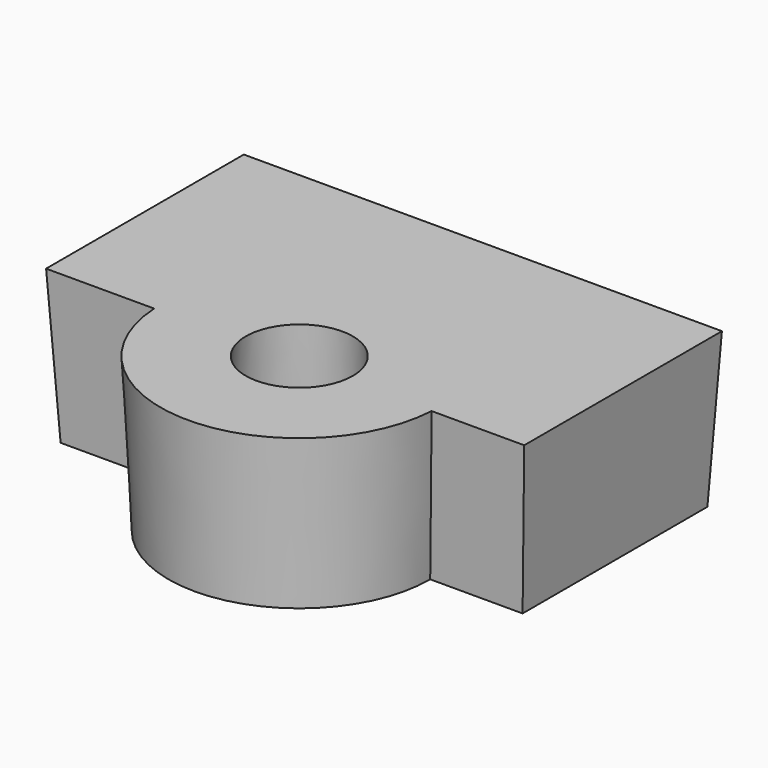
from build123d import *

# Parameters (mm, degrees)
F0_R                   = 10.16
F1_DEPTH               = 25.4
DRAFT_F1_DRAFTED_ANGLE = -3


# Not quite as in the source:
# - an extrude with a draft is written as a straight extrude whose walls are then drafted


with BuildPart() as f1:
    # F0 (on Top) → F1 (new body)
    with BuildSketch(Plane.XY):
        with BuildLine():
            Line((40.546802333, 18.3483660635), (-35.653197667, 18.3483660635))
            Line((-35.653197667, 18.3483660635), (-35.653197667, -19.7516339365))
            Line((-35.653197667, -19.7516339365), (-17.8675366967, -19.7516339365))
            ThreePointArc((-17.8675366967, -19.7516339365), (3.7196328181, -41.3388034514), (25.306802333, -19.7516339365))
            Line((25.306802333, -19.7516339365), (40.546802333, -19.7516339365))
            Line((40.546802333, -19.7516339365), (40.546802333, 18.3483660635))
        make_face()
        with Locations((3.7196328181, -19.7516339365)):
            Circle(F0_R, mode=Mode.SUBTRACT)
    extrude(amount=F1_DEPTH)

    # draft_F1_drafted
    draft_f1_drafted_walls = [f1.faces().sort_by_distance(p)[0] for p in [
        (40.546802333, -0.7016339365, 16.9333333333),
        (2.446802333, 18.3483660635, 16.9333333333),
        (-35.653197667, -0.7016339365, 16.9333333333),
        (-26.7603671819, -19.7516339365, 16.9333333333),
        (3.7196328181, -41.3388034514, 16.9333333333),
        (32.926802333, -19.7516339365, 16.9333333333),
        (-6.4403671819, -19.7516339365, 16.9333333333),
    ]]
    draft(draft_f1_drafted_walls, neutral_plane=Plane.XY, angle=DRAFT_F1_DRAFTED_ANGLE)


solid = f1.part
